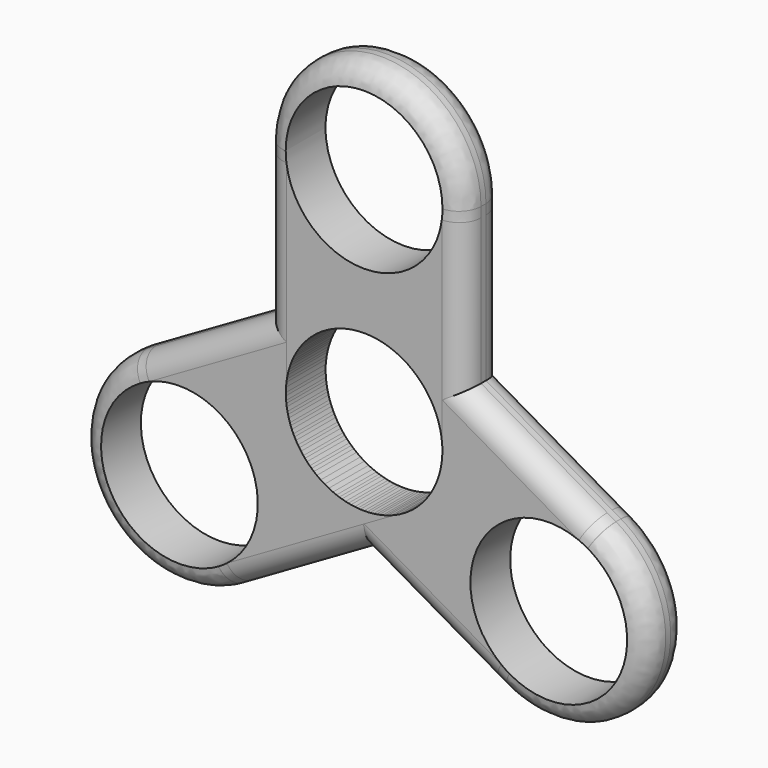
from build123d import *

# Parameters (mm, degrees)
F1_DEPTH        = 3.5
F1_COPIES_COUNT = 3
F3_R            = 3.0660512242
F3_2_R          = 3.0660512242
F3_3_R          = 3.0660512242


# Not quite as in the source:
# - a feature of the source that left no trace in its solid (it failed there, or was rolled back) is left out
# - a pattern or mirror of a feature is missing from the dataset's text; its kind, count and spacing are read off the source's solid


with BuildPart() as f1:
    # F0 (on Front) → F1 (new body, symmetric)
    with BuildSketch(Plane.XZ):
        with BuildLine():
            Line((14, -15), (14, 15))
            ThreePointArc((14, 15), (0, 1), (-14, 15))
            Line((-14, 15), (-14, -15))
            ThreePointArc((-14, -15), (0, -1), (14, -15))
        make_face()
        with BuildLine():
            ThreePointArc((-14, 15), (0, 1), (14, 15))
            Line((14, 15), (11.025, 15))
            ThreePointArc((11.025, 15), (0, 3.975), (-11.025, 15))
            Line((-11.025, 15), (-14, 15))
        make_face()
        with BuildLine():
            Line((11.025, 15), (14, 15))
            ThreePointArc((14, 15), (0, 29), (-14, 15))
            Line((-14, 15), (-11.025, 15))
            ThreePointArc((-11.025, 15), (0, 26.025), (11.025, 15))
        make_face()
        with BuildLine():
            ThreePointArc((-14, -15), (0, -29), (14, -15))
            Line((14, -15), (11.025, -15))
            ThreePointArc((11.025, -15), (0, -26.025), (-11.025, -15))
            Line((-11.025, -15), (-14, -15))
        make_face()
        with BuildLine():
            Line((11.025, -15), (14, -15))
            ThreePointArc((14, -15), (0, -1), (-14, -15))
            Line((-14, -15), (-11.025, -15))
            ThreePointArc((-11.025, -15), (0, -3.975), (11.025, -15))
        make_face()
    extrude(amount=F1_DEPTH, both=True)


with BuildPart() as f1_copies_1:
    # F1_copies: instance of F1
    add(f1.part.rotate(Axis((0, 0, -15), (0, 1, 0)), 1 * 360 / F1_COPIES_COUNT))

    # F3#2
    f3_2_edges = [f1_copies_1.edges().sort_by_distance(p)[0] for p in [
        (19.990381, 3.5, -10.375644),
        (19.990381, -3.5, -10.375644),
        (5.990381, 3.5, -34.624356),
        (5.990381, -3.5, -34.624356),
    ]]
    fillet(f3_2_edges, radius=F3_2_R)


with BuildPart() as f1_copies_2:
    # F1_copies: instance of F1
    add(f1.part.rotate(Axis((0, 0, -15), (0, 1, 0)), 2 * 360 / F1_COPIES_COUNT))

    # F3#3
    f3_3_edges = [f1_copies_2.edges().sort_by_distance(p)[0] for p in [
        (-5.990381, 3.5, -34.624356),
        (-5.990381, -3.5, -34.624356),
        (-19.990381, 3.5, -10.375644),
        (-19.990381, -3.5, -10.375644),
    ]]
    fillet(f3_3_edges, radius=F3_3_R)


with BuildPart() as f1_1:
    add(f1.part)

    # F3
    f3_edges = [f1_1.edges().sort_by_distance(p)[0] for p in [
        (14, 3.5, 0),
        (-14, 3.5, 0),
        (0, 3.5, 29),
        (-14, -3.5, 0),
        (0, -3.5, 29),
        (14, -3.5, 0),
    ]]
    fillet(f3_edges, radius=F3_R)


solid = Compound([f1_copies_1.part, f1_copies_2.part, f1_1.part])
